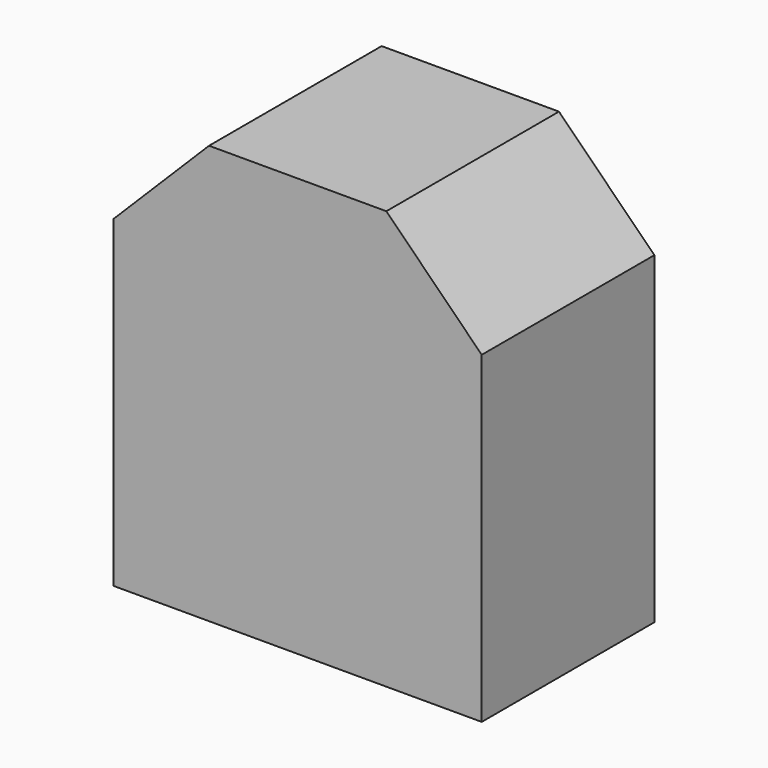
from build123d import *

# Parameters (mm, degrees)
F0_W     = 98.028793931
F0_H     = 57.4665814638
F1_DEPTH = 25.4
F2_SIZE  = 25.39999
F3_SIZE  = 25.39999
F4_DEPTH = 86.0725715756


# Not quite as in the source:
# - a fillet or chamfer is up to 0.001 mm smaller than in the source, because OpenCascade refuses the exact size


with BuildPart() as f1:
    # F0 (on Top) → F1 (new body)
    with BuildSketch(Plane.XY):
        with Locations((1.7422363162, 28.7332907319)):
            Rectangle(F0_W, F0_H)
    extrude(amount=F1_DEPTH)

    # F2 (size 25.4 in the source; OpenCascade refuses exactly that, so slightly less here)
    f2_edges = [f1.edges().sort_by_distance(p)[0] for p in [
        (50.756633, 28.733291, 25.4),
    ]]
    chamfer(f2_edges, length=F2_SIZE)

    # F3 (size 25.4 in the source; OpenCascade refuses exactly that, so slightly less here)
    f3_edges = [f1.edges().sort_by_distance(p)[0] for p in [
        (-47.272161, 28.733291, 25.4),
    ]]
    chamfer(f3_edges, length=F3_SIZE)

    # F4 (add): a face of the model
    f4_faces = [f1.faces().sort_by_distance(p)[0] for p in [
        (1.7422363162, 28.7332907319, 0),
    ]]
    extrude(f4_faces, amount=F4_DEPTH)


solid = f1.part
